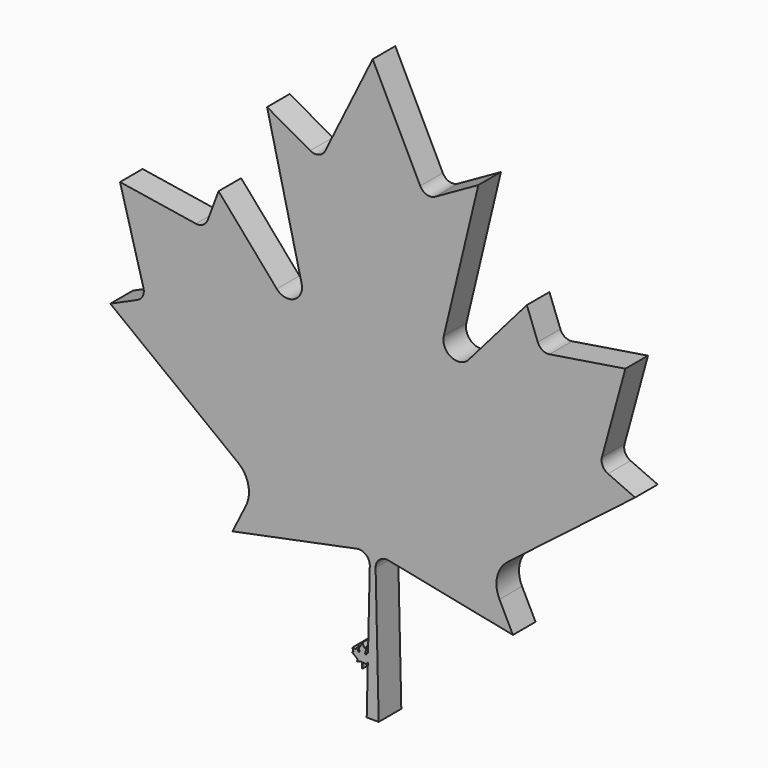
from build123d import *

# Parameters (mm, degrees)
F1_DEPTH = 1


# Not quite as in the source:
# - ends of sketch curves that miss each other by under 0.0002 mm in the source are joined


with BuildPart() as f1:
    # F0 (on Front) → F1 (new body)
    with BuildSketch(Plane.XZ):
        with BuildLine():
            Line((0.0528919554, 0.676734003), (-0.0133260446, 0.810837003))
            Line((-0.0133260446, 0.810837003), (-0.0133260446, 0.000355003))
            Line((-0.0133260446, 0.000355003), (-0.0049730446, 0.000355003))
            Line((-0.0049730446, 0.000355003), (-0.0092700446, 0.187913003))
            ThreePointArc((-0.0092700446, 0.187913003), (-0.0039052307, 0.1997565793), (0.0086959613, 0.2029600321))
            Line((0.0086959613, 0.2029600321), (0.1777903392, 0.168795789))
            Line((0.1777903392, 0.168795789), (0.1779611806, 0.1762527791))
            Line((0.1779611806, 0.1762527791), (0.1633489554, 0.205464003))
            ThreePointArc((0.1633489554, 0.205464003), (0.1601341311, 0.2322960931), (0.1747150055, 0.255048938))
            Line((0.1747150055, 0.255048938), (0.1798571632, 0.2590097465))
            Line((0.1798571632, 0.2590097465), (0.1868000755, 0.5620580937))
            Line((0.1868000755, 0.5620580937), (0.1202859554, 0.485431003))
            ThreePointArc((0.1202859554, 0.485431003), (0.0960352028, 0.4807561402), (0.0857322231, 0.5032011784))
            Line((0.0857322231, 0.5032011784), (0.1338759554, 0.704181003))
            Line((0.1338759554, 0.704181003), (0.0737009554, 0.670304003))
            ThreePointArc((0.0737009554, 0.670304003), (0.0619135468, 0.669043597), (0.0528919554, 0.676734003))
        make_face()
        with BuildLine():
            Line((-0.0133260446, 0.000355003), (-0.0133260446, 0.810837003))
            Line((-0.0133260446, 0.810837003), (-0.0795450446, 0.676734003))
            ThreePointArc((-0.0795450446, 0.676734003), (-0.0885662197, 0.6690437257), (-0.1003531884, 0.6703037475))
            Line((-0.1003531884, 0.6703037475), (-0.1605290446, 0.704181003))
            Line((-0.1605290446, 0.704181003), (-0.1123850446, 0.503201003))
            ThreePointArc((-0.1123850446, 0.503201003), (-0.1226883956, 0.4807560869), (-0.1469384945, 0.4854314805))
            Line((-0.1469384945, 0.4854314805), (-0.2281400446, 0.578978003))
            Line((-0.2281400446, 0.578978003), (-0.2433770446, 0.538362003))
            ThreePointArc((-0.2433770446, 0.538362003), (-0.2498706649, 0.5306698392), (-0.2597650019, 0.5288152727))
            Line((-0.2597650019, 0.5288152727), (-0.3654970446, 0.545543003))
            Line((-0.3654970446, 0.545543003), (-0.3328600446, 0.426430003))
            ThreePointArc((-0.3328600446, 0.426430003), (-0.3337663691, 0.4160544447), (-0.3412100188, 0.4087699453))
            Line((-0.3412100188, 0.4087699453), (-0.3790200446, 0.391884003))
            Line((-0.3790200446, 0.391884003), (-0.2013670446, 0.255049003))
            ThreePointArc((-0.2013670446, 0.255049003), (-0.1867871318, 0.232295707), (-0.1900021575, 0.2054640595))
            Line((-0.1900021575, 0.2054640595), (-0.2087830446, 0.167919003))
            Line((-0.2087830446, 0.167919003), (-0.0353490446, 0.202960003))
            ThreePointArc((-0.0353490446, 0.202960003), (-0.0227478586, 0.1997565793), (-0.0173829897, 0.1879130018))
            Line((-0.0173829897, 0.1879130018), (-0.0216800446, 0.000355003))
            Line((-0.0216800446, 0.000355003), (-0.0133260446, 0.000355003))
        make_face()
        Polygon((0.1779611806, 0.1762527791), (0.1777903392, 0.168795789), (0.1821299554, 0.167919003), align=None)
        Polygon((0.1821299554, 0.167919003), (0.1777903392, 0.168795789), (0.1401753438, -1.4730457961), (0.3523669438, -1.4730457961), (0.3523669438, 0.391884003), (0.1798571632, 0.2590097465), (0.1779611806, 0.1762527791), align=None)
        with BuildLine():
            Line((0.2493191438, 3.2909274039), (0.1868000755, 0.5620580937))
            Line((0.1868000755, 0.5620580937), (0.2014869554, 0.578978003))
            Line((0.2014869554, 0.578978003), (0.2167249554, 0.538362003))
            ThreePointArc((0.2167249554, 0.538362003), (0.2232185757, 0.5306698392), (0.2331129127, 0.5288152727))
            Line((0.2331129127, 0.5288152727), (0.3388449554, 0.545543003))
            Line((0.3388449554, 0.545543003), (0.3062069554, 0.426430003))
            ThreePointArc((0.3062069554, 0.426430003), (0.3071132799, 0.4160544447), (0.3145569296, 0.4087699453))
            Line((0.3145569296, 0.4087699453), (0.3523669554, 0.391884003))
            Line((0.3523669554, 0.391884003), (0.3523669438, 19.1131970039))
            Line((0.3523669438, 19.1131970039), (-1.3295956562, 15.7069808039))
            ThreePointArc((-1.3295956562, 15.7069808039), (-1.5587335044, 15.5116477594), (-1.858122509, 15.5436523149))
            Line((-1.858122509, 15.5436523149), (-3.3865892562, 16.4041346039))
            Line((-3.3865892562, 16.4041346039), (-2.1637316562, 11.2992426039))
            ThreePointArc((-2.1637316562, 11.2992426039), (-2.4254367706, 10.7291417351), (-3.0413892842, 10.8478967322))
            Line((-3.0413892842, 10.8478967322), (-5.1039086562, 13.2239784039))
            Line((-5.1039086562, 13.2239784039), (-5.4909284562, 12.1923320039))
            ThreePointArc((-5.4909284562, 12.1923320039), (-5.6558664119, 11.996951044), (-5.9071825723, 11.9498450545))
            Line((-5.9071825723, 11.9498450545), (-8.5927764562, 12.3747294039))
            Line((-8.5927764562, 12.3747294039), (-7.7637966562, 9.3492592039))
            ThreePointArc((-7.7637966562, 9.3492592039), (-7.786817298, 9.0857200238), (-7.9758860019, 8.9006937389))
            Line((-7.9758860019, 8.9006937389), (-8.9362606562, 8.4717908039))
            Line((-8.9362606562, 8.4717908039), (-4.4238744562, 4.9961818039))
            ThreePointArc((-4.4238744562, 4.9961818039), (-4.0535446709, 4.4182480852), (-4.1352063244, 3.7367242387))
            Line((-4.1352063244, 3.7367242387), (-4.6122408562, 2.7830798039))
            Line((-4.6122408562, 2.7830798039), (-0.2070172562, 3.6731212039))
            ThreePointArc((-0.2070172562, 3.6731212039), (0.1130528694, 3.5917542423), (0.2493191438, 3.2909274039))
        make_face()
        with BuildLine():
            Line((0.2014869554, 0.578978003), (0.1868000755, 0.5620580937))
            Line((0.1868000755, 0.5620580937), (0.1798571632, 0.2590097465))
            Line((0.1798571632, 0.2590097465), (0.3523669554, 0.391884003))
            Line((0.3523669554, 0.391884003), (0.3145569554, 0.408770003))
            ThreePointArc((0.3145569554, 0.408770003), (0.3071132799, 0.4160544447), (0.3062071928, 0.426429938))
            Line((0.3062071928, 0.426429938), (0.3388449554, 0.545543003))
            Line((0.3388449554, 0.545543003), (0.2331129554, 0.528815003))
            ThreePointArc((0.2331129554, 0.528815003), (0.2232185757, 0.5306698392), (0.2167248398, 0.5383619597))
            Line((0.2167248398, 0.5383619597), (0.2014869554, 0.578978003))
        make_face()
        with BuildLine():
            Line((0.3523669438, 0.391884003), (0.3523669438, -1.4730457961))
            Line((0.3523669438, -1.4730457961), (0.5645331438, -1.4730457961))
            Line((0.5645331438, -1.4730457961), (0.4553893438, 3.2909274039))
            ThreePointArc((0.4553893438, 3.2909274039), (0.5916556183, 3.5917542423), (0.9117258932, 3.6731219434))
            Line((0.9117258932, 3.6731219434), (5.3169493438, 2.7830798039))
            Line((5.3169493438, 2.7830798039), (4.8399119438, 3.7367228039))
            ThreePointArc((4.8399119438, 3.7367228039), (4.7582554065, 4.4182578922), (5.1286096155, 4.9961801528))
            Line((5.1286096155, 4.9961801528), (9.6409691438, 8.4717908039))
            Line((9.6409691438, 8.4717908039), (8.6805951438, 8.9006952039))
            ThreePointArc((8.6805951438, 8.9006952039), (8.4915257857, 9.0857200238), (8.4685111742, 9.3492575516))
            Line((8.4685111742, 9.3492575516), (9.2975103438, 12.3747294039))
            Line((9.2975103438, 12.3747294039), (6.6119175438, 11.9498382039))
            ThreePointArc((6.6119175438, 11.9498382039), (6.3606002996, 11.996951044), (6.1956594084, 12.1923309026))
            Line((6.1956594084, 12.1923309026), (5.8086171438, 13.2239784039))
            Line((5.8086171438, 13.2239784039), (3.7461117438, 10.8478846039))
            ThreePointArc((3.7461117438, 10.8478846039), (3.1301426273, 10.7291430881), (2.8684469448, 11.2992470593))
            Line((2.8684469448, 11.2992470593), (4.0912977438, 16.4041346039))
            Line((4.0912977438, 16.4041346039), (2.5628527438, 15.5436588039))
            ThreePointArc((2.5628527438, 15.5436588039), (2.2634525656, 15.511644492), (2.0343082289, 15.7069828209))
            Line((2.0343082289, 15.7069828209), (0.3523669438, 19.1131970039))
            Line((0.3523669438, 19.1131970039), (0.3523669438, 0.391884003))
        make_face()
    extrude(amount=F1_DEPTH)


solid = f1.part
